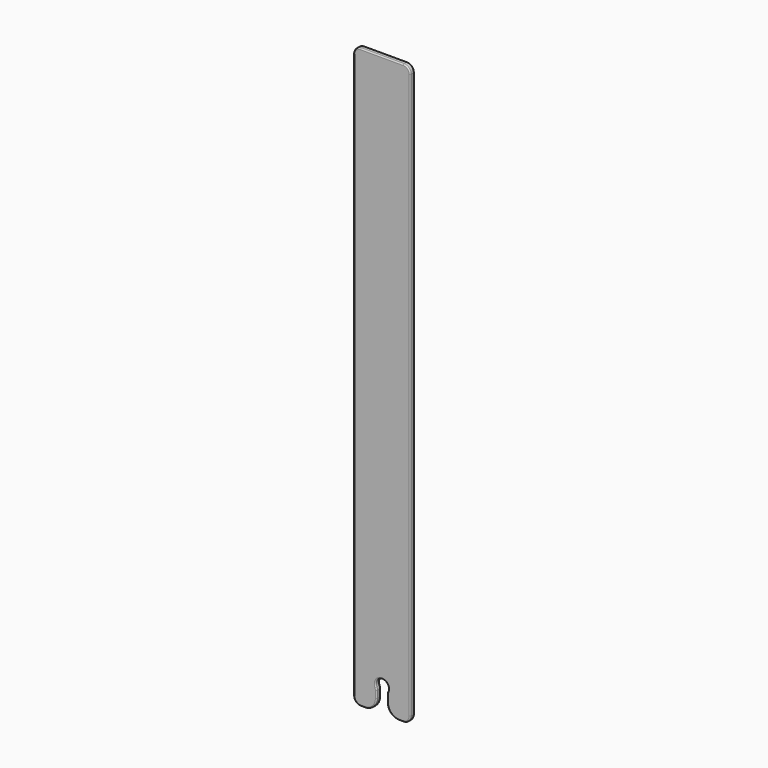
from build123d import *

# Parameters (mm, degrees)
F0_W          = 24
F0_H          = 2.2
F1_DEPTH      = 245
F3_DEPTH      = 1.101
F3_DEPTH_BACK = 1.101
F4_R          = 5
F5_R          = 3
F6_R          = 3
F7_R          = 0.5


with BuildPart() as f1:
    # F0 (on Top) → F1 (new body)
    with BuildSketch(Plane.XY):
        Rectangle(F0_W, F0_H)
    extrude(amount=F1_DEPTH)

    # F2 (on Front) → F3 (cut, two sides)
    with BuildSketch(Plane.XZ) as f3_sk:
        with BuildLine():
            Line((2.25, 0), (2.25, 8.6688611699))
            ThreePointArc((2.25, 8.6688611699), (0, 13), (-2.25, 8.6688611699))
            Line((-2.25, 8.6688611699), (-2.25, 0))
            Line((-2.25, 0), (2.25, 0))
        make_face()
    extrude(amount=-F3_DEPTH, mode=Mode.SUBTRACT)
    extrude(f3_sk.sketch, amount=F3_DEPTH_BACK, mode=Mode.SUBTRACT)

    # F4
    f4_edges = [f1.edges().sort_by_distance(p)[0] for p in [
        (2.25, 0, 0),
        (-2.25, 0, 0),
    ]]
    fillet(f4_edges, radius=F4_R)

    # F5
    f5_edges = [f1.edges().sort_by_distance(p)[0] for p in [
        (-2.25, 0, 8.668861),
        (2.25, 0, 8.668861),
    ]]
    fillet(f5_edges, radius=F5_R)

    # F6
    f6_edges = [f1.edges().sort_by_distance(p)[0] for p in [
        (12, 0, 245),
        (-12, 0, 245),
        (-12, 0, 0),
        (12, 0, 0),
    ]]
    fillet(f6_edges, radius=F6_R)

    # F7
    f7_edges = [f1.edges().sort_by_distance(p)[0] for p in [
        (-8.125, -1.1, 0),
        (-11.12132, -1.1, 0.87868),
        (-3.714466, -1.1, 1.464466),
        (-12, -1.1, 122.5),
        (-2.25, -1.1, 6.452396),
        (-11.12132, -1.1, 244.12132),
        (-2.315942, -1.1, 8.530335),
        (0, -1.1, 245),
        (0, -1.1, 13),
        (11.12132, -1.1, 244.12132),
        (2.315942, -1.1, 8.530335),
        (12, -1.1, 122.5),
        (2.25, -1.1, 6.452396),
        (11.12132, -1.1, 0.87868),
        (3.714466, -1.1, 1.464466),
        (8.125, -1.1, 0),
        (-8.125, 1.1, 0),
        (-11.12132, 1.1, 0.87868),
        (-3.714466, 1.1, 1.464466),
        (-12, 1.1, 122.5),
        (-2.25, 1.1, 6.452396),
        (-11.12132, 1.1, 244.12132),
        (-2.315942, 1.1, 8.530335),
        (0, 1.1, 245),
        (0, 1.1, 13),
        (11.12132, 1.1, 244.12132),
        (2.315942, 1.1, 8.530335),
        (12, 1.1, 122.5),
        (2.25, 1.1, 6.452396),
        (11.12132, 1.1, 0.87868),
        (3.714466, 1.1, 1.464466),
        (8.125, 1.1, 0),
    ]]
    fillet(f7_edges, radius=F7_R)


solid = f1.part
